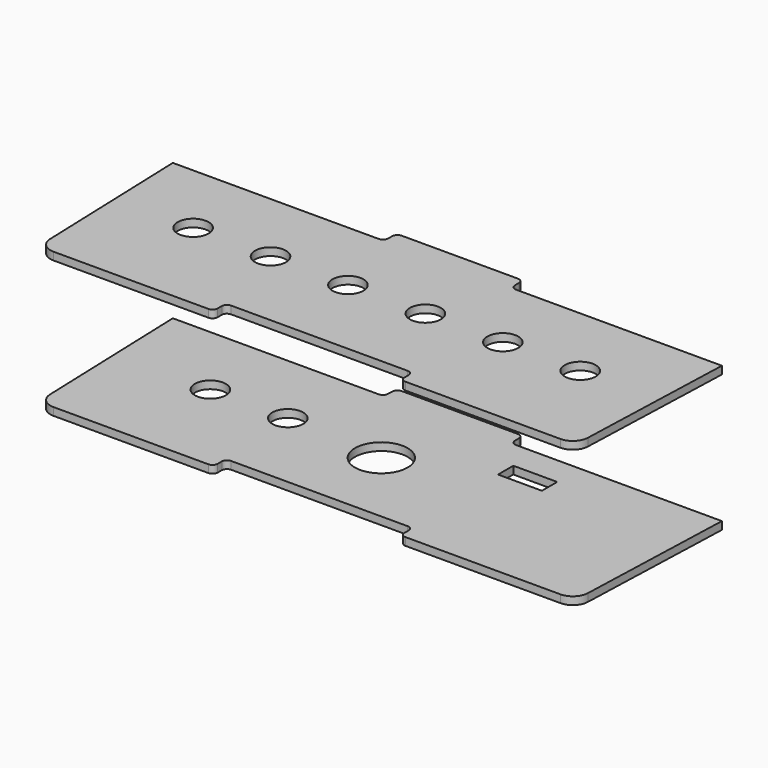
from build123d import *

# Parameters (mm, degrees)
F1_DEPTH = 1.5
F2_R     = 3
F2_R_2   = 5.1
F2_W     = 8.5
F2_H     = 3.7
F3_DEPTH = 25
F6_DEPTH = 1.5
F7_R     = 3
F8_DEPTH = 5


# Not quite as in the source:
# - ends of sketch curves that miss each other by under 0.0002 mm in the source are joined


with BuildPart() as f1:
    # F0 (on Top) → F1 (new body)
    with BuildSketch(Plane.XY):
        with BuildLine():
            ThreePointArc((49.102934, -18.5), (51.1869092815, -17.6580192367), (52.1011064976, -15.6046980174))
            Line((52.1011064976, -15.6046980174), (53.187306, 15.5))
            Line((53.187306, 15.5), (13.294894, 15.5))
            ThreePointArc((13.294894, 15.5), (12.6002354488, 15.7806603742), (12.2955031554, 16.4651010054))
            Line((12.2955031554, 16.4651010054), (12.258145, 17.534899))
            ThreePointArc((12.258145, 17.534899), (11.9534125512, 18.2193396258), (11.258754, 18.5))
            Line((11.258754, 18.5), (-11.258754, 18.5))
            ThreePointArc((-11.258754, 18.5), (-11.9534125512, 18.2193396258), (-12.2581448446, 17.5348989946))
            Line((-12.2581448446, 17.5348989946), (-12.295503, 16.465101))
            ThreePointArc((-12.295503, 16.465101), (-12.6002354488, 15.7806603742), (-13.294894, 15.5))
            Line((-13.294894, 15.5), (-53.187306, 15.5))
            Line((-53.187306, 15.5), (-52.101106, -15.604698))
            ThreePointArc((-52.101106, -15.604698), (-51.1869092815, -17.6580192367), (-49.102934, -18.5))
            Line((-49.102934, -18.5), (-19.10173, -18.5))
            ThreePointArc((-19.10173, -18.5), (-18.3946232188, -18.2071067812), (-18.10173, -17.5))
            Line((-18.10173, -17.5), (-18.10173, -16.5))
            ThreePointArc((-18.10173, -16.5), (-17.8088367812, -15.7928932188), (-17.10173, -15.5))
            Line((-17.10173, -15.5), (17.10173, -15.5))
            ThreePointArc((17.10173, -15.5), (17.8088367812, -15.7928932188), (18.10173, -16.5))
            Line((18.10173, -16.5), (18.10173, -17.5))
            ThreePointArc((18.10173, -17.5), (18.3946232188, -18.2071067812), (19.10173, -18.5))
            Line((19.10173, -18.5), (49.102934, -18.5))
        make_face()
    extrude(amount=F1_DEPTH)

    # F2 (on face) → F3 (cut)
    with BuildSketch(Plane.XY):
        with Locations((-34.155, 0.8)):
            Circle(F2_R)
        with Locations((-19.155, 0.8)):
            Circle(F2_R)
        with Locations((0, -0.5)):
            Circle(F2_R_2)
        with Locations((21.465, 8.1)):
            Rectangle(F2_W, F2_H)
    extrude(amount=F3_DEPTH, mode=Mode.SUBTRACT)


with BuildPart() as f6:
    # F5 (on offset) → F6 (new body)
    with BuildSketch(Plane.XY.offset(26.5)):
        with BuildLine():
            ThreePointArc((49.102934, -18.5), (51.1869092815, -17.6580192367), (52.1011064976, -15.6046980174))
            Line((52.1011064976, -15.6046980174), (53.187306, 15.5))
            Line((53.187306, 15.5), (13.294894, 15.5))
            ThreePointArc((13.294894, 15.5), (12.6002354488, 15.7806603742), (12.2955031554, 16.4651010054))
            Line((12.2955031554, 16.4651010054), (12.258145, 17.534899))
            ThreePointArc((12.258145, 17.534899), (11.9534125512, 18.2193396258), (11.258754, 18.5))
            Line((11.258754, 18.5), (-11.258754, 18.5))
            ThreePointArc((-11.258754, 18.5), (-11.9534125512, 18.2193396258), (-12.2581448446, 17.5348989946))
            Line((-12.2581448446, 17.5348989946), (-12.295503, 16.465101))
            ThreePointArc((-12.295503, 16.465101), (-12.6002354488, 15.7806603742), (-13.294894, 15.5))
            Line((-13.294894, 15.5), (-53.187306, 15.5))
            Line((-53.187306, 15.5), (-52.101106, -15.604698))
            ThreePointArc((-52.101106, -15.604698), (-51.1869092815, -17.6580192367), (-49.102934, -18.5))
            Line((-49.102934, -18.5), (-19.10173, -18.5))
            ThreePointArc((-19.10173, -18.5), (-18.3946232188, -18.2071067812), (-18.10173, -17.5))
            Line((-18.10173, -17.5), (-18.10173, -16.5))
            ThreePointArc((-18.10173, -16.5), (-17.8088367812, -15.7928932188), (-17.10173, -15.5))
            Line((-17.10173, -15.5), (17.10173, -15.5))
            ThreePointArc((17.10173, -15.5), (17.8088367812, -15.7928932188), (18.10173, -16.5))
            Line((18.10173, -16.5), (18.10173, -17.5))
            ThreePointArc((18.10173, -17.5), (18.3946232188, -18.2071067812), (19.10173, -18.5))
            Line((19.10173, -18.5), (49.102934, -18.5))
        make_face()
    extrude(amount=F6_DEPTH)

    # F7 (on face) → F8 (cut)
    with BuildSketch(Plane.XY.offset(28)):
        with Locations((-37.5, 0.8)):
            Circle(F7_R)
        with Locations((-22.5, 0.8)):
            Circle(F7_R)
        with Locations((-7.5, 0.8)):
            Circle(F7_R)
        with Locations((7.5, 0.8)):
            Circle(F7_R)
        with Locations((37.5, 0.8)):
            Circle(F7_R)
        with Locations((22.5, 0.8)):
            Circle(F7_R)
    extrude(amount=-F8_DEPTH, mode=Mode.SUBTRACT)


solid = Compound([f1.part, f6.part])
